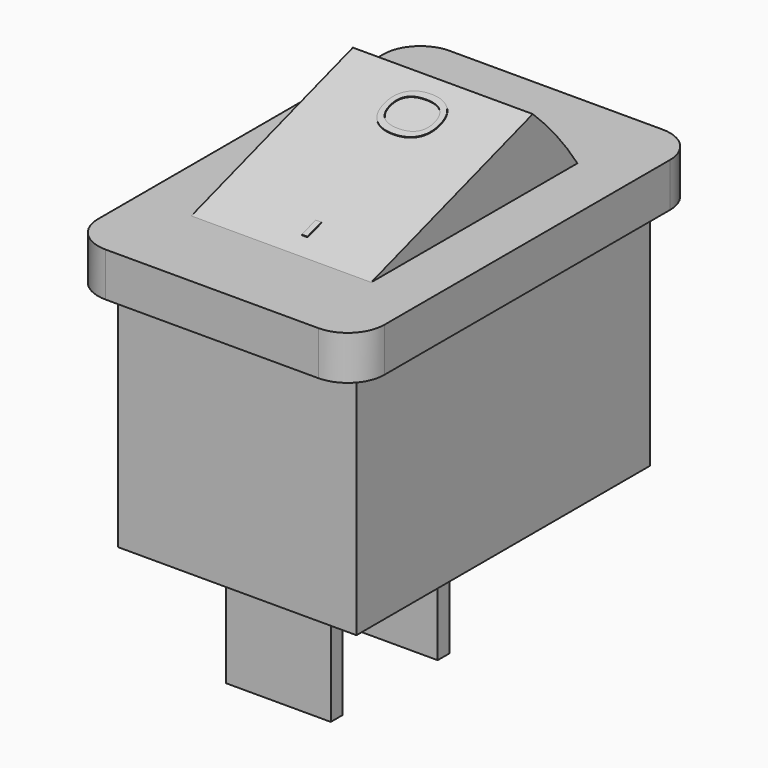
from build123d import *

# Parameters (mm, degrees)
F0_W          = 8.255
F0_H          = 12.7
F1_DEPTH      = 8.128
F2_W          = 9.906
F2_H          = 14.8844
F3_DEPTH      = 1.524
F6_DEPTH      = 6.223
F7_R          = 1.27
F8_W          = 3.6322
F8_H          = 0.508
F9_DEPTH      = 4.1148
F10_TEXT_SIZE = 2.6418773971
F11_DEPTH     = 0.0254


# Not quite as in the source:
# - Text() gives the source's letters only with a copy of the font that has no kerning and outlines rounded to 1/6400 em; it was checked with that copy


with BuildPart() as f1:
    # F0 (on Top) → F1 (new body)
    with BuildSketch(Plane.XY):
        with Locations((4.1275, 6.35)):
            Rectangle(F0_W, F0_H)
    extrude(amount=F1_DEPTH)

    # F2 (on face) → F3 (join)
    with BuildSketch(Plane.XY.offset(8.128)):
        with Locations((4.1275, 6.35)):
            Rectangle(F2_W, F2_H)
    extrude(amount=F3_DEPTH)

    # F5 (on offset) → F6 (join)
    with BuildSketch(Plane.YZ.offset(7.2517)):
        with BuildLine():
            Line((8.8773, 11.938), (1.8923, 9.652))
            Line((1.8923, 9.652), (10.8077, 9.652))
            ThreePointArc((10.8077, 9.652), (9.9100558322, 10.8520471472), (8.8773, 11.938))
        make_face()
    extrude(amount=-F6_DEPTH)

    # F7
    f7_edges = [f1.edges().sort_by_distance(p)[0] for p in [
        (9.0805, -1.0922, 8.89),
        (9.0805, 13.7922, 8.89),
        (-0.8255, 13.7922, 8.89),
        (-0.8255, -1.0922, 8.89),
    ]]
    fillet(f7_edges, radius=F7_R)

    # F8 (on face) → F9 (join)
    with BuildSketch(Plane(origin=(0, 0, 0), x_dir=(1, 0, 0), z_dir=(0, 0, -1))):
        with Locations((4.1275, -2.032)):
            Rectangle(F8_W, F8_H)
        with Locations((4.1275, -6.6548)):
            Rectangle(F8_W, F8_H)
    extrude(amount=F9_DEPTH)

    # F10 (on face) → F11 (join)
    with BuildSketch(Plane(origin=(0, -2.6701626754, 8.1588303971), x_dir=(1, 0, 0), z_dir=(0, -0.3110390604, 0.950397129))):
        with Locations(Location((5.1344376152, 5.3855211659), (0, 0, 90))):
            Text('-     O', F10_TEXT_SIZE, font='Open Sans', text_align=(TextAlign.LEFT, TextAlign.BOTTOM))
    extrude(amount=F11_DEPTH)


solid = f1.part
